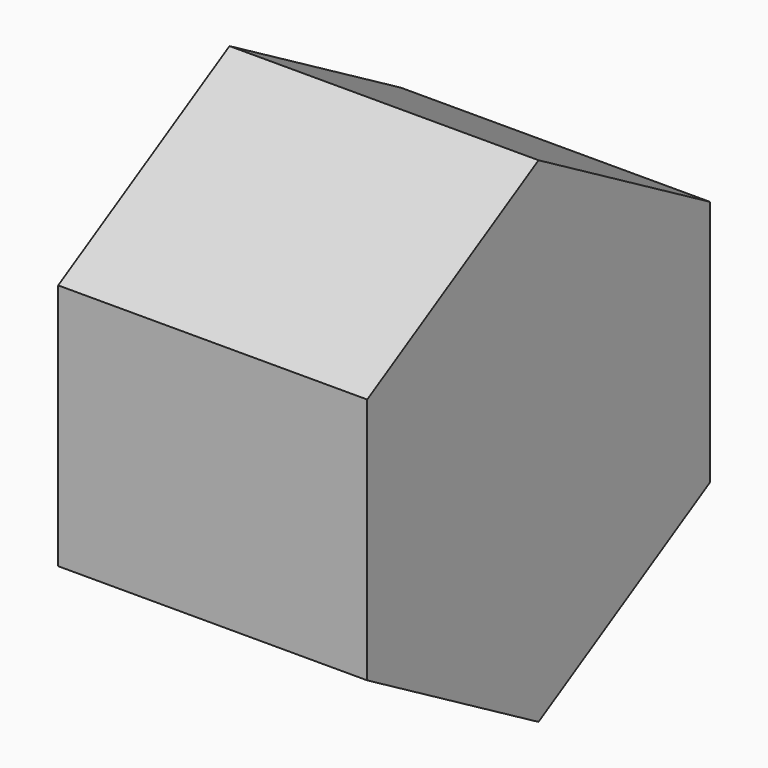
from build123d import *

# Parameters (mm, degrees)
F4_DEPTH = 25


# Not quite as in the source:
# - a feature of the source that left no trace in its solid (it failed there, or was rolled back) is left out
# - the program builds the solid bodies; features that only make, move or delete a surface that nothing else refers to are left out


with BuildPart() as f4:
    # F3 (on face) → F4 (new body)
    with BuildSketch(Plane.YZ.offset(100)):
        Polygon((17.3205080757, 10), (0, 20), (-17.3205080757, 10), (-17.3205080757, -10), (0, -20), (17.3205080757, -10), align=None)
    extrude(amount=F4_DEPTH)


solid = f4.part
